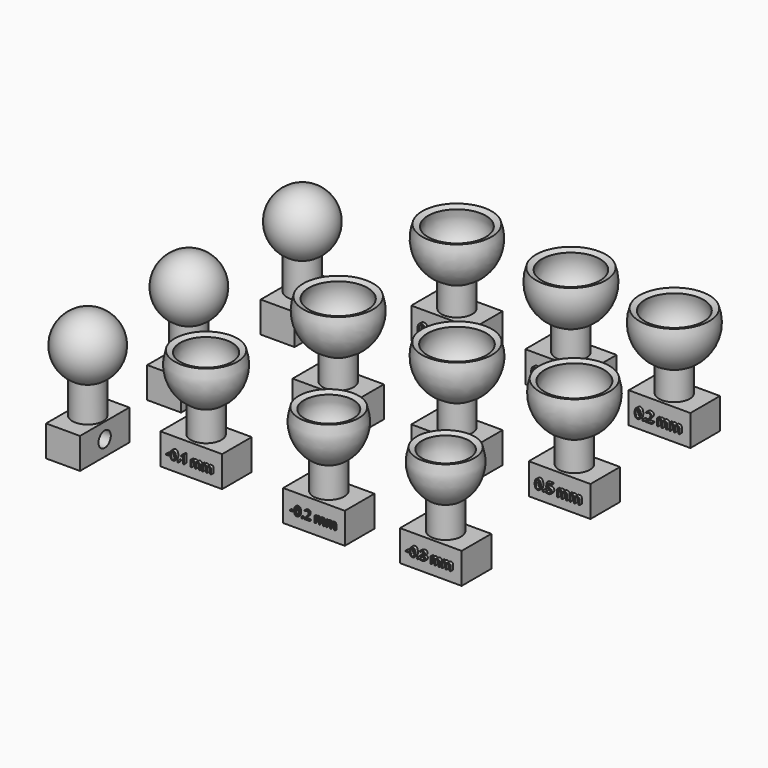
from build123d import *

# Parameters (mm, degrees)
F2_DEPTH      = 5.5
F3_ANGLE      = 90
F9_DEPTH      = 6
F10_TEXT_SIZE = 5.6061667835
F11_DEPTH     = 1
F14_DEPTH     = 6
F15_TEXT_SIZE = 4.2693231344
F16_DEPTH     = 1
F19_DEPTH     = 6
F20_TEXT_SIZE = 4.2693231344
F21_DEPTH     = 1
F24_DEPTH     = 6
F27_DEPTH     = 6
F30_DEPTH     = 6
F33_DEPTH     = 6
F36_DEPTH     = 6
F39_DEPTH     = 6
F40_TEXT_SIZE = 4.2693231344
F41_DEPTH     = 1
F42_TEXT_SIZE = 4.2693231344
F43_DEPTH     = 1
F44_TEXT_SIZE = 4.2693231344
F45_DEPTH     = 1
F46_TEXT_SIZE = 3.9111835404
F47_DEPTH     = 1
F48_TEXT_SIZE = 3.9111835404
F49_DEPTH     = 0.5
F50_TEXT_SIZE = 3.9111835404
F51_DEPTH     = 1
F52_ANGLE     = 90
F53_ANGLE     = 90
F54_ANGLE     = 90
F55_ANGLE     = 90
F56_ANGLE     = 90
F57_ANGLE     = 90
F58_ANGLE     = 90
F59_ANGLE     = 90
F60_ANGLE     = 90
F62_R         = 2.5
F63_DEPTH     = 25


# Not quite as in the source:
# - a feature names something its author has since deleted; it is built from what else it names
# - Text() gives the source's letters only with a copy of the font that has no kerning and outlines rounded to 1/6400 em; it was checked with that copy


with BuildPart() as f1:
    # F0 (on Top) → F1 (revolve)
    with BuildSketch(Plane.XY):
        with BuildLine():
            Line((-43.461524262, 53.6280996922), (-54.8012702242, 53.6280996922))
            Line((-54.8012702242, 53.6280996922), (-54.8012702242, 48.6280996922))
            Line((-54.8012702242, 48.6280996922), (-44.8012702242, 48.6280996922))
            ThreePointArc((-44.8012702242, 48.6280996922), (-44.4605284871, 51.2162901432), (-43.461524262, 53.6280996922))
        make_face()
        with BuildLine():
            ThreePointArc((-24.8012702242, 48.6280996922), (-32.2130797731, 58.2873579551), (-43.461524262, 53.6280996922))
            ThreePointArc((-43.461524262, 53.6280996922), (-44.4605284871, 51.2162901432), (-44.8012702242, 48.6280996922))
            Line((-44.8012702242, 48.6280996922), (-24.8012702242, 48.6280996922))
        make_face()
    revolve(axis=Axis((-34.8012702242, 48.6280996922, 0), (1, 0, 0)))

    # F0 (on Top) → F2 (join, symmetric)
    with BuildSketch(Plane.XY):
        Polygon((-54.8012702242, 53.6280996922), (-54.8012702242, 58.6280996922), (-64.8012702242, 58.6280996922), (-64.8012702242, 38.6280996922), (-54.8012702242, 38.6280996922), (-54.8012702242, 48.6280996922), align=None)
    extrude(amount=F2_DEPTH, both=True)


with BuildPart() as f1_1:
    # F3: moved
    add(f1.part.rotate(Axis((-64.8012702242, 48.6280996922, 0), (0, -1, 0)), F3_ANGLE))


with BuildPart() as f4_1:
    # F4: copy of F1
    add(f1_1.part.moved(Location((0, -20, 0))))


with BuildPart() as f4_1_1:
    # F5: moved
    add(f4_1.part.moved(Location((0, -20, 0))))


with BuildPart() as f6_1:
    # F6: copy of F4_1
    add(f4_1_1.part.moved(Location((0, -40, 0))))


with BuildPart() as f8:
    # F7 (on Top) → F8 (revolve)
    with BuildSketch(Plane.XY):
        with BuildLine():
            Line((-26.2671032548, 72.2231717465), (-26.2671032548, 69.9713155166))
            ThreePointArc((-26.2671032548, 69.9713155166), (-23.8266938469, 69.1493400904), (-21.2671032548, 68.8669614792))
            Line((-21.2671032548, 68.8669614792), (-21.2671032548, 70.8669614792))
            ThreePointArc((-21.2671032548, 70.8669614792), (-23.8564536375, 71.2156546299), (-26.2671032548, 72.2231717465))
        make_face()
        with BuildLine():
            Line((-26.2671032548, 69.9713155166), (-26.2671032548, 60.8669614792))
            Line((-26.2671032548, 60.8669614792), (-21.2671032548, 60.8669614792))
            Line((-21.2671032548, 60.8669614792), (-21.2671032548, 68.8669614792))
            ThreePointArc((-21.2671032548, 68.8669614792), (-23.8266938469, 69.1493400904), (-26.2671032548, 69.9713155166))
        make_face()
        with BuildLine():
            ThreePointArc((-32.5149565787, 84.9712147661), (-32.3161193981, 76.2528882886), (-26.2671032548, 69.9713155166))
            Line((-26.2671032548, 69.9713155166), (-26.2671032548, 72.2231717465))
            ThreePointArc((-26.2671032548, 72.2231717465), (-30.641192092, 77.4622111716), (-30.6355776931, 84.2871767929))
            Line((-30.6355776931, 84.2871767929), (-32.5149565787, 84.9712147661))
        make_face()
    revolve(axis=Axis((-21.2671032548, 65.8669614792, 0), (0, -1, 0)))

    # F7 (on Top) → F9 (join, symmetric)
    with BuildSketch(Plane.XY):
        Polygon((-26.2671032548, 60.8669614792), (-31.2671032548, 60.8669614792), (-31.2671032548, 50.8669614792), (-11.2671032548, 50.8669614792), (-11.2671032548, 60.8669614792), (-21.2671032548, 60.8669614792), align=None)
    extrude(amount=F9_DEPTH, both=True)

    # F10 (on face) → F11 (join)
    with BuildSketch(Plane.XY.offset(6)):
        with Locations((-28.7671032548, 53.3305213951)):
            Text('0 mm', F10_TEXT_SIZE, font='Open Sans', text_align=(TextAlign.LEFT, TextAlign.BOTTOM))
    extrude(amount=F11_DEPTH)


with BuildPart() as f13:
    # F12 (on Top) → F13 (revolve)
    with BuildSketch(Plane.XY):
        with BuildLine():
            ThreePointArc((4.9134033306, 84.3829168971), (5.1235516854, 75.6032002447), (11.2366994111, 69.2978840978))
            Line((11.2366994111, 69.2978840978), (11.2366994111, 71.5436328993))
            ThreePointArc((11.2366994111, 71.5436328993), (6.7977308498, 76.810723188), (6.7927885722, 83.6988766105))
            Line((6.7927885722, 83.6988766105), (4.9134033306, 84.3829168971))
        make_face()
        with BuildLine():
            Line((11.2366994111, 71.5436328993), (11.2366994111, 69.2978840978))
            ThreePointArc((11.2366994111, 69.2978840978), (13.678376266, 68.4862829768), (16.2366994111, 68.21157417))
            Line((16.2366994111, 68.21157417), (16.2366994111, 70.21157417))
            ThreePointArc((16.2366994111, 70.21157417), (13.6495010973, 70.5502969685), (11.2366994111, 71.5436328993))
        make_face()
        with BuildLine():
            Line((11.2366994111, 69.2978840978), (11.2366994111, 60.21157417))
            Line((11.2366994111, 60.21157417), (16.2366994111, 60.21157417))
            Line((16.2366994111, 60.21157417), (16.2366994111, 68.21157417))
            ThreePointArc((16.2366994111, 68.21157417), (13.678376266, 68.4862829768), (11.2366994111, 69.2978840978))
        make_face()
    revolve(axis=Axis((16.2366994111, 65.21157417, 0), (0, -1, 0)))

    # F12 (on Top) → F14 (join, symmetric)
    with BuildSketch(Plane.XY):
        Polygon((11.2366994111, 60.21157417), (6.2366994111, 60.21157417), (6.2366994111, 50.21157417), (26.2366994111, 50.21157417), (26.2366994111, 60.21157417), (16.2366994111, 60.21157417), align=None)
    extrude(amount=F14_DEPTH, both=True)

    # F15 (on face) → F16 (join)
    with BuildSketch(Plane.XY.offset(6)):
        with Locations((8.7366994111, 53.6376615133)):
            Text('0.1 mm', F15_TEXT_SIZE, font='Open Sans', text_align=(TextAlign.LEFT, TextAlign.BOTTOM))
    extrude(amount=F16_DEPTH)


with BuildPart() as f18:
    # F17 (on Top) → F18 (revolve)
    with BuildSketch(Plane.XY):
        with BuildLine():
            ThreePointArc((39.4089849459, 83.2271552801), (39.6442198767, 74.4699640229), (45.7482646406, 68.186304921))
            Line((45.7482646406, 68.186304921), (45.7482646406, 70.3244608214))
            ThreePointArc((45.7482646406, 70.3244608214), (41.2672648819, 75.6185235261), (41.2573691706, 82.5543984408))
            Line((41.2573691706, 82.5543984408), (39.4089849459, 83.2271552801))
        make_face()
        with BuildLine():
            Line((45.7482646406, 70.3244608214), (45.7482646406, 68.186304921))
            ThreePointArc((45.7482646406, 68.186304921), (48.1899414955, 67.3747038), (50.7482646406, 67.0999949932))
            Line((50.7482646406, 67.0999949932), (50.7482646406, 68.9999949932))
            ThreePointArc((50.7482646406, 68.9999949932), (48.1620410554, 69.3367246616), (45.7482646406, 70.3244608214))
        make_face()
        with BuildLine():
            Line((45.7482646406, 68.186304921), (45.7482646406, 58.9999949932))
            Line((45.7482646406, 58.9999949932), (50.7482646406, 58.9999949932))
            Line((50.7482646406, 58.9999949932), (50.7482646406, 67.0999949932))
            ThreePointArc((50.7482646406, 67.0999949932), (48.1899414955, 67.3747038), (45.7482646406, 68.186304921))
        make_face()
    revolve(axis=Axis((50.7482646406, 63.9999949932, 0), (0, -1, 0)))

    # F17 (on Top) → F19 (join, symmetric)
    with BuildSketch(Plane.XY):
        Polygon((45.7482646406, 58.9999949932), (40.7482646406, 58.9999949932), (40.7482646406, 48.9999949932), (60.7482646406, 48.9999949932), (60.7482646406, 58.9999949932), (50.7482646406, 58.9999949932), align=None)
    extrude(amount=F19_DEPTH, both=True)

    # F20 (on face) → F21 (join)
    with BuildSketch(Plane.XY.offset(6)):
        with Locations((43.2482646406, 52.4260823364)):
            Text('0.2 mm', F20_TEXT_SIZE, font='Open Sans', text_align=(TextAlign.LEFT, TextAlign.BOTTOM))
    extrude(amount=F21_DEPTH)


with BuildPart() as f23:
    # F22 (on Top) → F23 (revolve)
    with BuildSketch(Plane.XY):
        with BuildLine():
            ThreePointArc((-31.0499881043, 35.0884500089), (-30.7903842517, 26.3658548556), (-24.7107084095, 20.1057748222))
            Line((-24.7107084095, 20.1057748222), (-24.7107084095, 22.1282551359))
            ThreePointArc((-24.7107084095, 22.1282551359), (-29.2337283985, 27.4492261847), (-29.2485885105, 34.4327941768))
            Line((-29.2485885105, 34.4327941768), (-31.0499881043, 35.0884500089))
        make_face()
        with BuildLine():
            Line((-24.7107084095, 22.1282551359), (-24.7107084095, 20.1057748222))
            ThreePointArc((-24.7107084095, 20.1057748222), (-22.2694894571, 19.29000613), (-19.7107084095, 19.0113161888))
            Line((-19.7107084095, 19.0113161888), (-19.7107084095, 20.811289722))
            ThreePointArc((-19.7107084095, 20.811289722), (-22.2959742518, 21.1460515423), (-24.7107084095, 22.1282551359))
        make_face()
        with BuildLine():
            Line((-24.7107084095, 20.1057748222), (-24.7107084095, 10.811289722))
            Line((-24.7107084095, 10.811289722), (-19.7107084095, 10.811289722))
            Line((-19.7107084095, 10.811289722), (-19.7107084095, 19.0113161888))
            ThreePointArc((-19.7107084095, 19.0113161888), (-22.2694894571, 19.29000613), (-24.7107084095, 20.1057748222))
        make_face()
    revolve(axis=Axis((-19.7107084095, 30.961289722, 0), (0, 1, 0)))

    # F22 (on Top) → F24 (join, symmetric)
    with BuildSketch(Plane.XY):
        Polygon((-24.7107084095, 10.811289722), (-29.7107084095, 10.811289722), (-29.7107084095, 0.811289722), (-9.7107084095, 0.811289722), (-9.7107084095, 10.811289722), (-19.7107084095, 10.811289722), align=None)
    extrude(amount=F24_DEPTH, both=True)

    # F40 (on face) → F41 (join)
    with BuildSketch(Plane.XY.offset(6)):
        with Locations((-27.2107084095, 4.2373770653)):
            Text('0.3 mm', F40_TEXT_SIZE, font='Open Sans', text_align=(TextAlign.LEFT, TextAlign.BOTTOM))
    extrude(amount=F41_DEPTH)


with BuildPart() as f26:
    # F25 (on Top) → F26 (revolve)
    with BuildSketch(Plane.XY):
        with BuildLine():
            Line((14.4538154081, 19.4026113482), (14.4538154081, 10))
            Line((14.4538154081, 10), (19.4538154081, 10))
            Line((19.4538154081, 10), (19.4538154081, 18.3001044554))
            ThreePointArc((19.4538154081, 18.3001044554), (16.8945816598, 18.5827258024), (14.4538154081, 19.4026113482))
        make_face()
        with BuildLine():
            Line((14.4538154081, 21.3095556916), (14.4538154081, 19.4026113482))
            ThreePointArc((14.4538154081, 19.4026113482), (16.8945816598, 18.5827258024), (19.4538154081, 18.3001044554))
            Line((19.4538154081, 18.3001044554), (19.4538154081, 20))
            ThreePointArc((19.4538154081, 20), (16.8694907327, 20.3328187423), (14.4538154081, 21.3095556916))
        make_face()
        with BuildLine():
            ThreePointArc((8.1145357133, 34.3271602869), (8.3983286425, 25.6391073471), (14.4538154081, 19.4026113482))
            Line((14.4538154081, 19.4026113482), (14.4538154081, 21.3095556916))
            ThreePointArc((14.4538154081, 21.3095556916), (9.8887859718, 26.6573721783), (9.868950676, 33.6886054619))
            Line((9.868950676, 33.6886054619), (8.1145357133, 34.3271602869))
        make_face()
    revolve(axis=Axis((19.4538154081, 30.2, 0), (0, 1, 0)))

    # F25 (on Top) → F27 (join, symmetric)
    with BuildSketch(Plane.XY):
        Polygon((14.4538154081, 10), (9.4538154081, 10), (9.4538154081, 0), (29.4538154081, 0), (29.4538154081, 10), (19.4538154081, 10), align=None)
    extrude(amount=F27_DEPTH, both=True)

    # F42 (on face) → F43 (join)
    with BuildSketch(Plane.XY.offset(6)):
        with Locations((11.9538154081, 3.4260873432)):
            Text('0.4 mm', F42_TEXT_SIZE, font='Open Sans', text_align=(TextAlign.LEFT, TextAlign.BOTTOM))
    extrude(amount=F43_DEPTH)


with BuildPart() as f29:
    # F28 (on Top) → F29 (revolve)
    with BuildSketch(Plane.XY):
        with BuildLine():
            ThreePointArc((43.9607159959, 37.1771599542), (44.2685189687, 28.5235943747), (50.2999956906, 22.3106861616))
            Line((50.2999956906, 22.3106861616), (50.2999956906, 24.1022345832))
            ThreePointArc((50.2999956906, 24.1022345832), (45.6929674104, 29.4768347365), (45.6681463275, 36.5557061364))
            Line((45.6681463275, 36.5557061364), (43.9607159959, 37.1771599542))
        make_face()
        with BuildLine():
            Line((50.2999956906, 24.1022345832), (50.2999956906, 22.3106861616))
            ThreePointArc((50.2999956906, 22.3106861616), (52.7403144618, 21.4867345484), (55.2999956906, 21.2002315413))
            Line((55.2999956906, 21.2002315413), (55.2999956906, 22.7999996673))
            ThreePointArc((55.2999956906, 22.7999996673), (52.7165960033, 23.1308996045), (50.2999956906, 24.1022345832))
        make_face()
        with BuildLine():
            Line((50.2999956906, 22.3106861616), (50.2999956906, 12.7999996673))
            Line((50.2999956906, 12.7999996673), (55.2999956906, 12.7999996673))
            Line((55.2999956906, 12.7999996673), (55.2999956906, 21.2002315413))
            ThreePointArc((55.2999956906, 21.2002315413), (52.7403144618, 21.4867345484), (50.2999956906, 22.3106861616))
        make_face()
    revolve(axis=Axis((55.2999956906, 33.0499996673, 0), (0, 1, 0)))

    # F28 (on Top) → F30 (join, symmetric)
    with BuildSketch(Plane.XY):
        Polygon((50.2999956906, 12.7999996673), (45.2999956906, 12.7999996673), (45.2999956906, 2.7999996673), (65.2999956906, 2.7999996673), (65.2999956906, 12.7999996673), (55.2999956906, 12.7999996673), align=None)
    extrude(amount=F30_DEPTH, both=True)

    # F44 (on face) → F45 (join)
    with BuildSketch(Plane.XY.offset(6)):
        with Locations((47.7999956906, 6.2260870106)):
            Text('0.5 mm', F44_TEXT_SIZE, font='Open Sans', text_align=(TextAlign.LEFT, TextAlign.BOTTOM))
    extrude(amount=F45_DEPTH)


with BuildPart() as f32:
    # F31 (on Top) → F32 (revolve)
    with BuildSketch(Plane.XY):
        with BuildLine():
            ThreePointArc((-33.7581096791, -13.9064893473), (-33.7600743796, -22.0481190748), (-28.5653088987, -28.3171341552))
            Line((-28.5653088987, -28.3171341552), (-28.5653088987, -25.9807123348))
            ThreePointArc((-28.5653088987, -25.9807123348), (-32.1510040666, -20.8315979833), (-31.9631177619, -14.5598129759))
            Line((-31.9631177619, -14.5598129759), (-33.7581096791, -13.9064893473))
        make_face()
        with BuildLine():
            Line((-28.5653088987, -25.9807123348), (-28.5653088987, -28.3171341552))
            ThreePointArc((-28.5653088987, -28.3171341552), (-26.1546595996, -29.4005699565), (-23.5653088987, -29.9300282896))
            Line((-23.5653088987, -29.9300282896), (-23.5653088987, -27.9300282896))
            ThreePointArc((-23.5653088987, -27.9300282896), (-26.1985145304, -27.2970430702), (-28.5653088987, -25.9807123348))
        make_face()
        with BuildLine():
            Line((-28.5653088987, -28.3171341552), (-28.5653088987, -37.9300282896))
            Line((-28.5653088987, -37.9300282896), (-23.5653088987, -37.9300282896))
            Line((-23.5653088987, -37.9300282896), (-23.5653088987, -29.9300282896))
            ThreePointArc((-23.5653088987, -29.9300282896), (-26.1546595996, -29.4005699565), (-28.5653088987, -28.3171341552))
        make_face()
    revolve(axis=Axis((-23.5653088987, -17.9800282896, 0), (0, 1, 0)))

    # F31 (on Top) → F33 (join, symmetric)
    with BuildSketch(Plane.XY):
        Polygon((-28.5653088987, -37.9300282896), (-33.5653088987, -37.9300282896), (-33.5653088987, -47.9300282896), (-13.5653088987, -47.9300282896), (-13.5653088987, -37.9300282896), (-23.5653088987, -37.9300282896), align=None)
    extrude(amount=F33_DEPTH, both=True)

    # F46 (on face) → F47 (join)
    with BuildSketch(Plane.XY.offset(6)):
        with Locations((-31.0653088987, -44.2460804387)):
            Text('-0.1 mm', F46_TEXT_SIZE, font='Open Sans', text_align=(TextAlign.LEFT, TextAlign.BOTTOM))
    extrude(amount=F47_DEPTH)


with BuildPart() as f35:
    # F34 (on Top) → F35 (revolve)
    with BuildSketch(Plane.XY):
        with BuildLine():
            ThreePointArc((6.1541429183, -13.5675617442), (6.0716660225, -21.4519506164), (10.900000222, -27.6855353944))
            Line((10.900000222, -27.6855353944), (10.900000222, -25.3029703915))
            ThreePointArc((10.900000222, -25.3029703915), (7.6545291294, -20.2271817321), (7.9139971371, -14.2080962965))
            Line((7.9139971371, -14.2080962965), (6.1541429183, -13.5675617442))
        make_face()
        with BuildLine():
            Line((10.900000222, -25.3029703915), (10.900000222, -27.6855353944))
            ThreePointArc((10.900000222, -27.6855353944), (13.296418865, -28.8879705339), (15.900000222, -29.5283116102))
            Line((15.900000222, -29.5283116102), (15.900000222, -27.5283116102))
            ThreePointArc((15.900000222, -27.5283116102), (13.2448018857, -26.7643478306), (10.900000222, -25.3029703915))
        make_face()
        with BuildLine():
            Line((10.900000222, -27.6855353944), (10.900000222, -37.5283116102))
            Line((10.900000222, -37.5283116102), (15.900000222, -37.5283116102))
            Line((15.900000222, -37.5283116102), (15.900000222, -29.5283116102))
            ThreePointArc((15.900000222, -29.5283116102), (13.296418865, -28.8879705339), (10.900000222, -27.6855353944))
        make_face()
    revolve(axis=Axis((15.900000222, -17.6283116102, 0), (0, 1, 0)))

    # F34 (on Top) → F36 (join, symmetric)
    with BuildSketch(Plane.XY):
        Polygon((10.900000222, -37.5283116102), (5.900000222, -37.5283116102), (5.900000222, -47.5283116102), (25.900000222, -47.5283116102), (25.900000222, -37.5283116102), (15.900000222, -37.5283116102), align=None)
    extrude(amount=F36_DEPTH, both=True)

    # F48 (on face) → F49 (join, symmetric)
    with BuildSketch(Plane.XY.offset(6)):
        with Locations((8.400000222, -43.8443637593)):
            Text('-0.2 mm', F48_TEXT_SIZE, font='Open Sans', text_align=(TextAlign.LEFT, TextAlign.BOTTOM))
    extrude(amount=F49_DEPTH, both=True)


with BuildPart() as f38:
    # F37 (on Top) → F38 (revolve)
    with BuildSketch(Plane.XY):
        with BuildLine():
            ThreePointArc((43.3407339979, -12.3121087052), (43.1986700002, -19.9934636564), (47.7447110415, -26.1867589761))
            Line((47.7447110415, -26.1867589761), (47.7447110415, -23.7633269899))
            ThreePointArc((47.7447110415, -23.7633269899), (44.7619007383, -18.7596965439), (45.073525268, -12.9427931497))
            Line((45.073525268, -12.9427931497), (43.3407339979, -12.3121087052))
        make_face()
        with BuildLine():
            Line((47.7447110415, -23.7633269899), (47.7447110415, -26.1867589761))
            ThreePointArc((47.7447110415, -26.1867589761), (50.1293650154, -27.4845130973), (52.7447110415, -28.2130084634))
            Line((52.7447110415, -28.2130084634), (52.7447110415, -26.2130084634))
            ThreePointArc((52.7447110415, -26.2130084634), (50.0707806037, -25.3431739583), (47.7447110415, -23.7633269899))
        make_face()
        with BuildLine():
            Line((47.7447110415, -26.1867589761), (47.7447110415, -36.2130084634))
            Line((47.7447110415, -36.2130084634), (52.7447110415, -36.2130084634))
            Line((52.7447110415, -36.2130084634), (52.7447110415, -28.2130084634))
            ThreePointArc((52.7447110415, -28.2130084634), (50.1293650154, -27.4845130973), (47.7447110415, -26.1867589761))
        make_face()
    revolve(axis=Axis((52.7447110415, -16.3630084634, 0), (0, 1, 0)))

    # F37 (on Top) → F39 (join, symmetric)
    with BuildSketch(Plane.XY):
        Polygon((47.7447110415, -36.2130084634), (42.7447110415, -36.2130084634), (42.7447110415, -46.2130084634), (62.7447110415, -46.2130084634), (62.7447110415, -36.2130084634), (52.7447110415, -36.2130084634), align=None)
    extrude(amount=F39_DEPTH, both=True)

    # F50 (on face) → F51 (join)
    with BuildSketch(Plane.XY.offset(6)):
        with Locations((45.2447110415, -42.5290606125)):
            Text('-0.3 mm', F50_TEXT_SIZE, font='Open Sans', text_align=(TextAlign.LEFT, TextAlign.BOTTOM))
    extrude(amount=F51_DEPTH)


with BuildPart() as f8_1:
    # F52: moved
    add(f8.part.rotate(Axis((-21.2671032548, 50.8669614792, 6), (1, 0, 0)), F52_ANGLE))


with BuildPart() as f13_1:
    # F53: moved
    add(f13.part.rotate(Axis((16.2366994111, 50.21157417, 6), (1, 0, 0)), F53_ANGLE))


with BuildPart() as f18_1:
    # F54: moved
    add(f18.part.rotate(Axis((50.7482646406, 48.9999949932, 6), (1, 0, 0)), F54_ANGLE))


with BuildPart() as f23_1:
    # F55: moved
    add(f23.part.rotate(Axis((-19.7107084095, 0.811289722, 6), (1, 0, 0)), F55_ANGLE))


with BuildPart() as f26_1:
    # F56: moved
    add(f26.part.rotate(Axis((19.4538154081, 0, 6), (1, 0, 0)), F56_ANGLE))


with BuildPart() as f29_1:
    # F57: moved
    add(f29.part.rotate(Axis((55.2999956906, 2.7999996673, 6), (1, 0, 0)), F57_ANGLE))


with BuildPart() as f32_1:
    # F58: moved
    add(f32.part.rotate(Axis((-23.5653088987, -47.9300282896, 6), (1, 0, 0)), F58_ANGLE))


with BuildPart() as f35_1:
    # F59: moved
    add(f35.part.rotate(Axis((15.900000222, -47.5283116102, 6), (1, 0, 0)), F59_ANGLE))


with BuildPart() as f38_1:
    # F60: moved
    add(f38.part.rotate(Axis((52.7447110415, -46.2130084634, 6), (1, 0, 0)), F60_ANGLE))


with BuildPart() as f32_2:
    # F61: moved
    add(f32_1.part.moved(Location((0, 0, 3.5))))


with BuildPart() as f1_2:
    add(f1_1.part)

    # F62 (on face) → F63 (cut)
    with BuildSketch(Plane(origin=(-70.3012702242, 0, 0), x_dir=(0, -1, 0), z_dir=(-1, 0, 0))):
        with Locations((-48.6280996922, 5)):
            Circle(F62_R)
    extrude(amount=-F63_DEPTH, mode=Mode.SUBTRACT)


with BuildPart() as f65_1:
    # F65: copy of F1
    add(f1_2.part.moved(Location((0, -46, 0))))


with BuildPart() as f66_1:
    # F66: copy of F65_1
    add(f65_1.part.moved(Location((0, -41, 0))))


solid = Compound([f8_1.part, f13_1.part, f18_1.part, f23_1.part, f26_1.part, f29_1.part, f35_1.part, f38_1.part, f32_2.part, f1_2.part, f65_1.part, f66_1.part])
